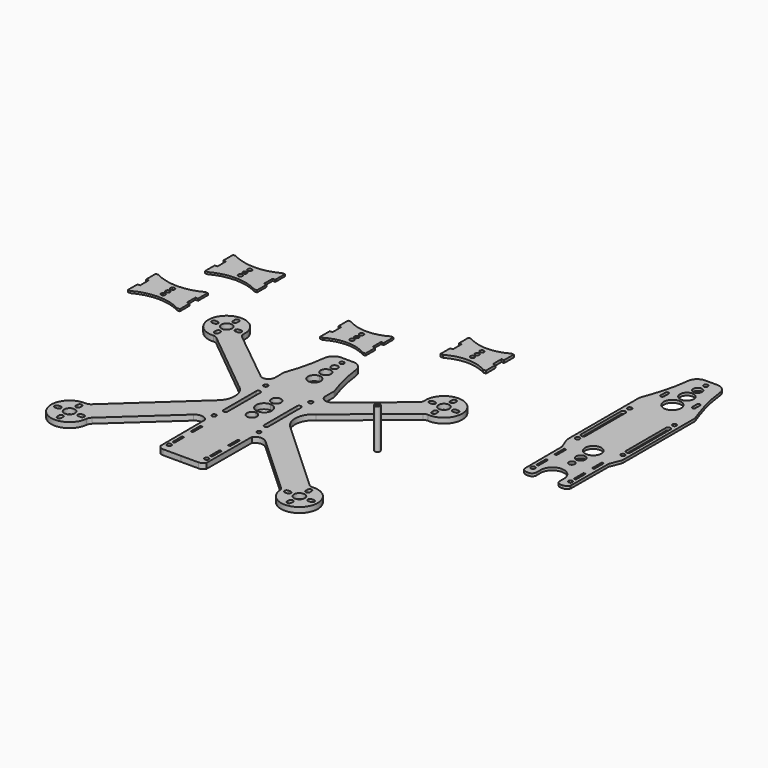
from build123d import *

# Parameters (mm, degrees)
F0_W      = 2
F0_H      = 9.1
F3_DEPTH  = 1.5
F4_W      = 2
F4_H      = 9.1
F5_DEPTH  = 2
F2_R      = 1.5875
F2_W      = 1.6002
F2_H      = 9.125
F6_DEPTH  = 2
F1_R      = 4
F1_R_2    = 1.5875
F7_DEPTH  = 4
F8_R      = 2
F8_R_2    = 1.3
F9_DEPTH  = 30
F10_W     = 2
F10_H     = 9.1
F11_DEPTH = 1.5
F12_W     = 2
F12_H     = 9.1
F13_DEPTH = 1.5


# Not quite as in the source:
# - ends of sketch curves that miss each other by under 0.0002 mm in the source are joined


with BuildPart() as f3:
    # F0 (on Top) → F3 (new body)
    with BuildSketch(Plane.XY):
        with BuildLine():
            Line((-44.4664459562, 44.7763409459), (-57.9039463685, 44.7763409459))
            Line((-57.9039463685, 44.7763409459), (-57.9039463685, 40.7740757426))
            Line((-57.9039463685, 40.7740757426), (-57.9039463685, 31.6763409459))
            ThreePointArc((-57.9039463685, 31.6763409459), (-42.9039463685, 35.7117386538), (-27.9039463685, 31.6763409459))
            Line((-27.9039463685, 31.6763409459), (-27.9039463685, 40.7740757426))
            Line((-27.9039463685, 40.7740757426), (-27.9039463685, 44.7763409459))
            Line((-27.9039463685, 44.7763409459), (-41.3414467807, 44.7763409459))
            ThreePointArc((-41.3414467807, 44.7763409459), (-41.7994933789, 43.6722203901), (-42.9039463685, 43.2149759459))
            ThreePointArc((-42.9039463685, 43.2149759459), (-44.0083993581, 43.6722203901), (-44.4664459562, 44.7763409459))
        make_face()
        with BuildLine():
            ThreePointArc((-42.9039463685, 38.8387946912), (-44.4664463685, 40.4012946912), (-42.9039463685, 41.9637946912))
            ThreePointArc((-42.9039463685, 41.9637946912), (-41.3414463685, 40.4012946912), (-42.9039463685, 38.8387946912))
        make_face(mode=Mode.SUBTRACT)
        with BuildLine():
            ThreePointArc((-27.9039463685, 57.8763409459), (-42.9039463685, 53.840943238), (-57.9039463685, 57.8763409459))
            Line((-57.9039463685, 57.8763409459), (-57.9039463685, 48.7763409459))
            Line((-57.9039463685, 48.7763409459), (-57.9039463685, 44.7763409459))
            Line((-57.9039463685, 44.7763409459), (-44.4664459562, 44.7763409459))
            ThreePointArc((-44.4664459562, 44.7763409459), (-44.0092019243, 45.8819289355), (-42.9039463685, 46.3399759459))
            ThreePointArc((-42.9039463685, 46.3399759459), (-41.7986908126, 45.8819289355), (-41.3414467807, 44.7763409459))
            Line((-41.3414467807, 44.7763409459), (-27.9039463685, 44.7763409459))
            Line((-27.9039463685, 44.7763409459), (-27.9039463685, 48.7763409459))
            Line((-27.9039463685, 48.7763409459), (-27.9039463685, 57.8763409459))
        make_face()
        with BuildLine():
            ThreePointArc((-42.9039463685, 50.8341467508), (-41.3414463685, 49.2716467508), (-42.9039463685, 47.7091467508))
            ThreePointArc((-42.9039463685, 47.7091467508), (-44.4664463685, 49.2716467508), (-42.9039463685, 50.8341467508))
        make_face(mode=Mode.SUBTRACT)
        with Locations((-26.9039463685, 53.3263409459)):
            Rectangle(F0_W, F0_H)
        Polygon((-25.9039463685, 40.7740757426), (-27.9039463685, 40.7740757426), (-27.9039463685, 31.6763409459), (-27.9039463685, 31.6740757426), (-25.9039463685, 31.6740757426), align=None)
        with Locations((-58.9039463685, 53.3263409459)):
            Rectangle(F0_W, F0_H)
        Polygon((-57.9039463685, 31.6763409459), (-57.9039463685, 40.7740757426), (-59.9039463685, 40.7740757426), (-59.9039463685, 31.6740757426), align=None)
    extrude(amount=F3_DEPTH)


with BuildPart() as f5:
    # F4 (on Top) → F5 (new body)
    with BuildSketch(Plane.XY):
        with BuildLine():
            ThreePointArc((41.3305214981, 84.1898763973), (26.3305214981, 80.1544786894), (11.3305214981, 84.1898763973))
            Line((11.3305214981, 84.1898763973), (11.3305214981, 75.0898763973))
            Line((11.3305214981, 75.0898763973), (11.3305214981, 71.0898763973))
            Line((11.3305214981, 71.0898763973), (24.7680219104, 71.0898763973))
            ThreePointArc((24.7680219104, 71.0898763973), (25.2252659423, 72.1954643869), (26.3305214981, 72.6535113973))
            ThreePointArc((26.3305214981, 72.6535113973), (27.435777054, 72.1954643869), (27.8930210859, 71.0898763973))
            Line((27.8930210859, 71.0898763973), (41.3305214981, 71.0898763973))
            Line((41.3305214981, 71.0898763973), (41.3305214981, 75.0898763973))
            Line((41.3305214981, 75.0898763973), (41.3305214981, 84.1898763973))
        make_face()
        with BuildLine():
            ThreePointArc((26.3305214981, 77.1476822022), (27.8930214981, 75.5851822022), (26.3305214981, 74.0226822022))
            ThreePointArc((26.3305214981, 74.0226822022), (24.7680214981, 75.5851822022), (26.3305214981, 77.1476822022))
        make_face(mode=Mode.SUBTRACT)
        with BuildLine():
            Line((24.7680219104, 71.0898763973), (11.3305214981, 71.0898763973))
            Line((11.3305214981, 71.0898763973), (11.3305214981, 67.087611194))
            Line((11.3305214981, 67.087611194), (11.3305214981, 57.9898763973))
            ThreePointArc((11.3305214981, 57.9898763973), (26.3305214981, 62.0252741052), (41.3305214981, 57.9898763973))
            Line((41.3305214981, 57.9898763973), (41.3305214981, 67.087611194))
            Line((41.3305214981, 67.087611194), (41.3305214981, 71.0898763973))
            Line((41.3305214981, 71.0898763973), (27.8930210859, 71.0898763973))
            ThreePointArc((27.8930210859, 71.0898763973), (27.4349744877, 69.9857558415), (26.3305214981, 69.5285113973))
            ThreePointArc((26.3305214981, 69.5285113973), (25.2260685085, 69.9857558415), (24.7680219104, 71.0898763973))
        make_face()
        with BuildLine():
            ThreePointArc((26.3305214981, 65.1523301426), (24.7680214981, 66.7148301426), (26.3305214981, 68.2773301426))
            ThreePointArc((26.3305214981, 68.2773301426), (27.8930214981, 66.7148301426), (26.3305214981, 65.1523301426))
        make_face(mode=Mode.SUBTRACT)
        Polygon((43.3305214981, 67.087611194), (41.3305214981, 67.087611194), (41.3305214981, 57.9898763973), (41.3305214981, 57.987611194), (43.3305214981, 57.987611194), align=None)
        with Locations((42.3305214981, 79.6398763973)):
            Rectangle(F4_W, F4_H)
        with Locations((10.3305214981, 79.6398763973)):
            Rectangle(F4_W, F4_H)
        Polygon((11.3305214981, 57.9898763973), (11.3305214981, 67.087611194), (9.3305214981, 67.087611194), (9.3305214981, 57.987611194), align=None)
    extrude(amount=F5_DEPTH)


with BuildPart() as f6:
    # F2 (on Top) → F6 (new body)
    with BuildSketch(Plane.XY):
        with BuildLine():
            Line((155.8763528676, 128.4774524202), (155.876246806, 128.4774524202))
            Line((155.876246806, 128.4774524202), (155.8761407443, 128.4774523998))
            Line((155.8761407443, 128.4774524202), (151.3094100886, 128.4774524202))
            ThreePointArc((151.3094100886, 128.4774524202), (146.4127010934, 126.6167403622), (143.9873656319, 121.9737072753))
            ThreePointArc((143.9873656319, 121.9737072753), (141.4366050173, 107.6108511655), (137.2573015197, 93.6347487897))
            Line((137.2573015197, 93.6347487897), (135.1935563122, 87.8591692184))
            ThreePointArc((135.1935563122, 87.8591692184), (135.0530988776, 87.3255692993), (135.0058168173, 86.7758224745))
            Line((135.0058168173, 86.7758224745), (135.0058168173, 19.9100591445))
            ThreePointArc((135.0058168173, 19.9100591445), (135.060963688, 19.3167136901), (135.2245151263, 18.743694552))
            Line((135.2245151263, 18.743694552), (138.1936514036, 11.1045397683))
            ThreePointArc((138.1936514036, 11.1045397683), (138.3556602367, 10.5396894348), (138.4123067823, 9.9548014711))
            Line((138.4123067823, 9.9548014711), (138.5925678775, -24.9512348722))
            ThreePointArc((138.5925678775, -24.9512348722), (140.1852851433, -26.826426264), (142.5436343491, -27.5273400025))
            Line((142.5436343491, -27.5273400025), (143.8996695078, -27.5273400025))
            ThreePointArc((143.8996695078, -27.5273400025), (146.1762594456, -26.5843455743), (147.1192538738, -24.3077556365))
            Line((147.1192538738, -24.3077556365), (147.1192538738, -20.6247556365))
            ThreePointArc((147.1192538738, -20.6247556365), (149.5794377566, -14.2301788079), (155.8897137171, -11.5611837055))
            ThreePointArc((155.8897137171, -11.5611837055), (162.2005028923, -14.2289650945), (164.6619166073, -20.6230686343))
            Line((164.6619166073, -20.6230686343), (164.6626249637, -24.3060685662))
            ThreePointArc((164.6626249637, -24.3060685662), (165.6060572341, -26.5824770945), (167.8828284972, -27.5250336456))
            Line((167.8828284972, -27.5250336456), (169.2388636308, -27.5247728375))
            ThreePointArc((169.2388636308, -27.5247728375), (171.5970779853, -26.8234055275), (173.1894345635, -24.9479078408))
            Line((173.1894345635, -24.9479078408), (173.3629821298, 9.9581625267))
            ThreePointArc((173.3629821298, 9.9581625267), (173.419516182, 10.5430613745), (173.5814163737, 11.1079428569))
            Line((173.5814163737, 11.1079428569), (176.5490833471, 18.7476685573))
            ThreePointArc((176.5490833471, 18.7476685573), (176.7125245728, 19.3207191409), (176.7675573235, 19.9140751908))
            Line((176.7675573235, 19.9140751908), (176.75469694, 86.7798372841))
            ThreePointArc((176.75469694, 86.7798372841), (176.707309147, 87.3295750049), (176.566749087, 87.8631478997))
            Line((176.566749087, 87.8631478997), (174.5018930926, 93.6383304413))
            ThreePointArc((174.5018930926, 93.6383304413), (170.3199016294, 107.6136287475), (167.7663786343, 121.9759940003))
            ThreePointArc((167.7663786343, 121.9759940003), (165.3401502168, 126.6185605332), (160.4430834388, 128.4783307661))
            Line((160.4430834388, 128.4783307661), (155.8763528676, 128.4774524405))
        make_face()
        with Locations((141.8560239264, -20.8835245555)):
            Circle(F2_R, mode=Mode.SUBTRACT)
        with Locations((141.8121739264, -12.3689241031)):
            Rectangle(F2_W, F2_H, mode=Mode.SUBTRACT)
        with Locations((141.8121739264, 4.7560758969)):
            Rectangle(F2_W, F2_H, mode=Mode.SUBTRACT)
        with Locations((138.9069576182, 24.590704959)):
            Circle(F2_R, mode=Mode.SUBTRACT)
        with BuildLine():
            ThreePointArc((137.3194112546, 67.0549892372), (139.055853514, 68.7740672747), (140.7575203822, 67.0205591086))
            Line((140.7575203822, 67.0205591086), (140.7578639328, 33.6104760546))
            Line((140.7578639328, 33.6104760546), (140.7578639328, 29.88865924))
            ThreePointArc((140.7578639328, 29.88865924), (139.0386515777, 28.1694424664), (137.3194303855, 29.8886504028))
            Line((137.3194303855, 29.8886504028), (137.3194112546, 33.6104406975))
            Line((137.3194112546, 33.6104406975), (137.3194112546, 67.0549892372))
        make_face(mode=Mode.SUBTRACT)
        with BuildLine():
            ThreePointArc((155.8890146168, -4.2914356483), (153.6566095072, -2.0721551798), (155.8885877383, 0.1475546091))
            ThreePointArc((155.8885877383, 0.1475546091), (158.1209928479, -2.0717258593), (155.8890146168, -4.2914356483))
        make_face(mode=Mode.SUBTRACT)
        with BuildLine():
            ThreePointArc((155.8883440274, 2.6818353952), (152.4370678505, 6.1205559329), (155.8876825898, 9.5599401956))
            ThreePointArc((155.8876825898, 9.5599401956), (159.3389587667, 6.1212196579), (155.8883440274, 2.6818353952))
        make_face(mode=Mode.SUBTRACT)
        with Locations((169.9251962268, -20.8808252644)):
            Circle(F2_R, mode=Mode.SUBTRACT)
        Polygon((170.7833763753, -7.7891995153), (170.7939351549, -16.9141934064), (169.1937362262, -16.9160450403), (169.1831774466, -7.7910511492), align=None, mode=Mode.SUBTRACT)
        Polygon((169.1633616547, 9.3339373861), (170.7635605834, 9.33578902), (170.774119363, 0.2107951289), (169.1739204343, 0.208943495), align=None, mode=Mode.SUBTRACT)
        with BuildLine():
            ThreePointArc((155.887452897, 11.9484512722), (149.8388017165, 17.9959392192), (155.8862896635, 24.0445903996))
            ThreePointArc((155.8862896635, 24.0445903996), (161.9349408439, 17.9971024527), (155.887452897, 11.9484512722))
        make_face(mode=Mode.SUBTRACT)
        with Locations((172.8655163598, 24.593970607)):
            Circle(F2_R, mode=Mode.SUBTRACT)
        with BuildLine():
            Line((174.4448954802, 67.0585594347), (174.4513279159, 33.6140115137))
            Line((174.4513279159, 33.6140115137), (174.452024602, 29.8922212841))
            ThreePointArc((174.452024602, 29.8922212841), (172.7331341001, 28.1726783007), (171.0135911167, 29.8915688027))
            Line((171.0135911167, 29.8915688027), (171.0128752946, 33.6133855484))
            Line((171.0128752946, 33.6133855484), (171.0067930382, 67.0234680505))
            ThreePointArc((171.0067930382, 67.0234680505), (172.7081226203, 68.7773034681), (174.4448954802, 67.0585594347))
        make_face(mode=Mode.SUBTRACT)
        with Locations((139.0386355169, 73.1351176697)):
            Circle(F2_R, mode=Mode.SUBTRACT)
        with BuildLine():
            ThreePointArc((145.2786560799, 101.8923559826), (145.2789936045, 101.8634246129), (145.2786560799, 101.8344932432))
            Line((145.2786560799, 101.8344932432), (145.2786560799, 97.5675112372))
            ThreePointArc((145.2786560799, 97.5675112372), (144.0533460411, 96.2985500188), (142.7987651392, 97.5385798675))
            Line((142.7987651392, 97.5385798675), (142.7987651392, 101.8634246129))
            ThreePointArc((142.7987651392, 101.8634246129), (144.0244127026, 103.1034544616), (145.2786560799, 101.8923559826))
        make_face(mode=Mode.SUBTRACT)
        with BuildLine():
            ThreePointArc((155.8803682862, 85.6193339205), (149.3345290592, 92.1782157718), (155.8791066864, 98.738356472))
            ThreePointArc((155.8791066864, 98.738356472), (162.4249459134, 92.1794746207), (155.8803682862, 85.6193339205))
        make_face(mode=Mode.SUBTRACT)
        with BuildLine():
            ThreePointArc((155.8789190085, 100.6899668871), (150.7560297607, 105.8118709374), (155.8779338109, 110.9347601852))
            ThreePointArc((155.8779338109, 110.9347601852), (161.0008230587, 105.8128561349), (155.8789190085, 100.6899668871))
        make_face(mode=Mode.SUBTRACT)
        with BuildLine():
            ThreePointArc((155.8777775383, 112.5597952039), (152.5637159996, 115.8732194059), (155.8771402016, 119.1872809446))
            ThreePointArc((155.8771402016, 119.1872809446), (159.1912017404, 115.8738567426), (155.8777775383, 112.5597952039))
        make_face(mode=Mode.SUBTRACT)
        with BuildLine():
            ThreePointArc((155.8776198499, 121.8899531092), (155.8768802972, 121.8899525924), (155.8761407443, 121.8899524202))
            ThreePointArc((155.8761407443, 121.8899524202), (154.2886407443, 123.4774524202), (155.8761407443, 125.0649524202))
            ThreePointArc((155.8761407443, 125.0649524202), (155.8765749713, 125.0649523608), (155.8770091982, 125.0649521826))
            ThreePointArc((155.8770091982, 125.0649521826), (157.464814495, 123.4777578591), (155.8776198499, 121.8899531092))
        make_face(mode=Mode.SUBTRACT)
        with Locations((172.7245018504, 73.1383570941)):
            Circle(F2_R, mode=Mode.SUBTRACT)
        with BuildLine():
            Line((166.4797822871, 97.569550058), (166.4789616126, 101.836531985))
            ThreePointArc((166.4789616126, 101.836531985), (166.4786185237, 101.8654632893), (166.4789504838, 101.8943947234))
            ThreePointArc((166.4789504838, 101.8943947234), (167.7329609058, 103.1057344103), (168.9588469431, 101.865940315))
            Line((168.9588469431, 101.865940315), (168.9596787464, 97.5410956496))
            ThreePointArc((168.9596787464, 97.5410956496), (167.7053363643, 96.3008245286), (166.4797822871, 97.569550058))
        make_face(mode=Mode.SUBTRACT)
    extrude(amount=F6_DEPTH)


with BuildPart() as f7:
    # F1 (on Top) → F7 (new body)
    with BuildSketch(Plane.XY):
        with BuildLine():
            Line((55.4423254621, -122.5938338167), (0.8312747552, -72.31776433))
            ThreePointArc((0.8312747552, -72.31776433), (-3.5713049649, -60.9524483755), (2.7441297756, -50.5280347721))
            Line((2.7441297756, -50.5280347721), (51.3242171863, -10.8932593465))
            ThreePointArc((51.3242171863, -10.8932593465), (52.7416112401, -10.1252404704), (54.3419180454, -9.9306202585))
            ThreePointArc((54.3419180454, -9.9306202585), (64.9351919977, 13.5546172758), (41.5501281912, 2.7420030758))
            ThreePointArc((41.5501281912, 2.7420030758), (41.2088558578, 0.7019316724), (39.9579419517, -0.945360814))
            Line((39.9579419517, -0.945360814), (0.7025146083, -32.6546178727))
            ThreePointArc((0.7025146083, -32.6546178727), (0.5270704544, -32.8033856058), (0.3447342931, -32.9436211712))
            ThreePointArc((0.3447342931, -32.9436211712), (-4.4980122119, -33.4435704761), (-7.3103707873, -29.4695571065))
            Line((-7.3103707873, -29.4695571065), (-7.3103707873, -21.2279371224))
            ThreePointArc((-7.3103707873, -21.2279371224), (-7.359671037, -20.6666688157), (-7.506061955, -20.1225894777))
            ThreePointArc((-7.506061955, -20.1225894777), (-11.7540587598, -6.0107609715), (-14.3386475919, 8.4981701128))
            ThreePointArc((-14.3386475919, 8.4981701128), (-16.7639830534, 13.1412031997), (-21.6606920486, 15.0019152577))
            Line((-21.6606920486, 15.0019152577), (-21.8785842975, 15.0019152577))
            Line((-21.8785842975, 15.0019152577), (-26.2273166427, 15.0019152577))
            Line((-26.2273166427, 15.0019152577), (-26.2274227043, 15.0019152577))
            Line((-26.2274227, 15.0019152577), (-26.2275287659, 15.0019152577))
            Line((-26.2275287659, 15.0019152578), (-30.5762611111, 15.0019211709))
            Line((-30.5762611111, 15.0019211709), (-30.7941533515, 15.0019214672))
            ThreePointArc((-30.7941533515, 15.0019214672), (-35.6908648767, 13.1412160673), (-38.1162066515, 8.4981862783))
            ThreePointArc((-38.1162066515, 8.4981862783), (-40.7008152117, -6.0107412918), (-44.9488312046, -20.1225640219))
            ThreePointArc((-44.9488312046, -20.1225640219), (-45.0952228624, -20.6666431607), (-45.1445238753, -21.2279114005))
            Line((-45.1445238753, -21.2279114005), (-45.1445350817, -29.4695313845))
            ThreePointArc((-45.1445350817, -29.4695313845), (-47.9568990637, -33.4435409315), (-52.7996448913, -32.9435850363))
            ThreePointArc((-52.7996448913, -32.9435850363), (-52.9819808591, -32.8033492249), (-53.157424808, -32.6545812554))
            Line((-53.1574248114, -32.6545812596), (-92.4128090441, -0.9452708203))
            ThreePointArc((-92.4128090441, -0.9452708203), (-93.6637207103, 0.7020233671), (-94.0049902698, 2.7420952345))
            ThreePointArc((-94.0049902698, 2.7420952345), (-117.3900393741, 13.5547412317), (-106.7967973552, -9.9305107065))
            ThreePointArc((-106.7967973552, -9.9305107065), (-105.1964908146, -10.1251330944), (-103.7790978051, -10.8931538978))
            Line((-103.7790978051, -10.8931538978), (-55.1990642866, -50.5279953787))
            ThreePointArc((-55.1990642866, -50.5279953787), (-48.8836437205, -60.9524175694), (-53.2862388943, -72.3177275376))
            Line((-53.2862388943, -72.3177275376), (-107.8973579627, -122.5937227683))
            ThreePointArc((-107.8973579627, -122.5937227683), (-109.6107464229, -123.6269577519), (-111.5920541618, -123.9056945287))
            ThreePointArc((-111.5920541618, -123.9056945287), (-122.9110206968, -146.5408303371), (-98.756834306, -138.9881052472))
            ThreePointArc((-98.756834306, -138.9881052472), (-98.2529376891, -137.2450612479), (-97.1601953583, -135.7966040057))
            Line((-97.1601953583, -135.7966040057), (-53.1895755998, -95.4842191234))
            ThreePointArc((-53.1895755998, -95.4842191234), (-48.3264853126, -93.815903761), (-43.7964935435, -96.2473843514))
            ThreePointArc((-43.7964935435, -96.2473843514), (-43.7450638141, -96.3412440629), (-43.7269025606, -96.446718379))
            Line((-43.7269025606, -96.446718379), (-43.51109813, -138.4267485338))
            ThreePointArc((-43.51109813, -138.4267485338), (-41.9183834139, -140.3019420913), (-39.5600351612, -141.0028590364))
            Line((-39.5600351612, -141.0028590364), (-26.2275287659, -141.0028771649))
            Line((-26.2275287659, -141.0028771649), (-12.8950223707, -141.0028771649))
            ThreePointArc((-12.8950223707, -141.0028771649), (-10.5366731649, -140.3019634265), (-8.9439558991, -138.4267720346))
            Line((-8.9439558991, -138.4267720346), (-8.7280943872, -96.4467421734))
            ThreePointArc((-8.7280943872, -96.4467421734), (-8.7099329903, -96.3412678819), (-8.6585031333, -96.2474082404))
            ThreePointArc((-8.6585031333, -96.2474082404), (-4.1285080581, -93.8159338094), (0.7345799607, -95.4842557844))
            Line((0.7345799607, -95.4842557844), (44.7051449055, -135.7967004544))
            ThreePointArc((44.7051449055, -135.7967004544), (45.7978852668, -137.2451591825), (46.3017795137, -138.988203867))
            ThreePointArc((46.3017795137, -138.988203867), (70.4559556348, -146.5409617999), (59.1370198774, -123.9058106008))
            ThreePointArc((59.1370198774, -123.9058106008), (57.1557125175, -123.62707113), (55.4423254621, -122.5938338167))
        make_face()
        with BuildLine():
            Line((-114.039597116, -147.1295236826), (-114.0395949405, -145.5295236826))
            ThreePointArc((-114.0395949405, -145.5295236826), (-112.4395927649, -143.9295258581), (-110.8395949405, -145.5295280337))
            Line((-110.8395949405, -145.5295280337), (-110.839597116, -147.1295280337))
            ThreePointArc((-110.839597116, -147.1295280337), (-112.4395992916, -148.7295258581), (-114.039597116, -147.1295236826))
        make_face(mode=Mode.SUBTRACT)
        with BuildLine():
            ThreePointArc((-122.0395863742, -139.2295128048), (-123.6395841987, -137.6295106292), (-122.0395820231, -136.0295128048))
            Line((-122.0395820231, -136.0295128048), (-120.4395820231, -136.0295149804))
            ThreePointArc((-120.4395820231, -136.0295149804), (-118.8395841987, -137.6295171559), (-120.4395863742, -139.2295149803))
            Line((-120.4395863742, -139.2295149803), (-122.0395863742, -139.2295128048))
        make_face(mode=Mode.SUBTRACT)
        with Locations((-112.4395841987, -137.6295258581)):
            Circle(F1_R, mode=Mode.SUBTRACT)
        with BuildLine():
            ThreePointArc((-104.4395863742, -139.2295367359), (-106.0395841987, -137.6295345604), (-104.4395820231, -136.0295367359))
            Line((-104.4395820231, -136.0295367359), (-102.8395820231, -136.0295389115))
            ThreePointArc((-102.8395820231, -136.0295389115), (-101.2395841987, -137.629541087), (-102.8395863742, -139.2295389115))
            Line((-102.8395863742, -139.2295389115), (-104.4395863742, -139.2295367359))
        make_face(mode=Mode.SUBTRACT)
        with BuildLine():
            ThreePointArc((-114.0395712813, -128.1295236826), (-112.4395691057, -126.5295258581), (-110.8395712813, -128.1295280337))
            Line((-110.8395712813, -128.1295280337), (-110.8395734569, -129.7295280337))
            ThreePointArc((-110.8395734569, -129.7295280337), (-112.4395756324, -131.3295258581), (-114.0395734569, -129.7295236826))
            Line((-114.0395734569, -129.7295236826), (-114.0395712813, -128.1295236826))
        make_face(mode=Mode.SUBTRACT)
        with Locations((-40.2476365481, -134.3575674396)):
            Circle(F1_R_2, mode=Mode.SUBTRACT)
        Polygon((-39.4913811763, -130.4069432304), (-41.0915811763, -130.4069410545), (-41.0915687689, -121.2819410546), (-39.4913687689, -121.2819432304), align=None, mode=Mode.SUBTRACT)
        Polygon((-39.4913578911, -113.2819432304), (-41.0915578911, -113.2819410546), (-41.0915454836, -104.1569410546), (-39.4913454836, -104.1569432304), align=None, mode=Mode.SUBTRACT)
        with Locations((-43.064958687, -88.83576076)):
            Circle(F1_R_2, mode=Mode.SUBTRACT)
        with Locations((-12.207411948, -134.357586503)):
            Circle(F1_R_2, mode=Mode.SUBTRACT)
        Polygon((-11.363488763, -121.2819410546), (-11.3634763555, -130.4069410545), (-12.9636763555, -130.4069432304), (-12.963688763, -121.2819432304), align=None, mode=Mode.SUBTRACT)
        with BuildLine():
            Line((58.3845312536, -147.1296430826), (58.3845312536, -145.5296430826))
            ThreePointArc((58.3845312536, -145.5296430826), (59.9845312536, -143.9296430826), (61.5845312536, -145.5296430826))
            Line((61.5845312536, -145.5296430826), (61.5845312536, -147.1296430826))
            ThreePointArc((61.5845312536, -147.1296430826), (59.9845312536, -148.7296430826), (58.3845312536, -147.1296430826))
        make_face(mode=Mode.SUBTRACT)
        with BuildLine():
            Line((50.3845312536, -136.0296430826), (51.9845312536, -136.0296430826))
            ThreePointArc((51.9845312536, -136.0296430826), (53.5845312536, -137.6296430826), (51.9845312536, -139.2296430826))
            Line((51.9845312536, -139.2296430826), (50.3845312536, -139.2296430826))
            ThreePointArc((50.3845312536, -139.2296430826), (48.7845312536, -137.6296430826), (50.3845312536, -136.0296430826))
        make_face(mode=Mode.SUBTRACT)
        with Locations((59.9845312536, -137.6296430826)):
            Circle(F1_R, mode=Mode.SUBTRACT)
        with BuildLine():
            Line((67.9845312536, -136.0296430826), (69.5845312536, -136.0296430826))
            ThreePointArc((69.5845312536, -136.0296430826), (71.1845312536, -137.6296430826), (69.5845312536, -139.2296430826))
            Line((69.5845312536, -139.2296430826), (67.9845312536, -139.2296430826))
            ThreePointArc((67.9845312536, -139.2296430826), (66.3845312536, -137.6296430826), (67.9845312536, -136.0296430826))
        make_face(mode=Mode.SUBTRACT)
        with BuildLine():
            Line((61.5845312536, -128.1296430826), (61.5845312536, -129.7296430826))
            ThreePointArc((61.5845312536, -129.7296430826), (59.9845312536, -131.3296430826), (58.3845312536, -129.7296430826))
            Line((58.3845312536, -129.7296430826), (58.3845312536, -128.1296430826))
            ThreePointArc((58.3845312536, -128.1296430826), (59.9845312536, -126.5296430826), (61.5845312536, -128.1296430826))
        make_face(mode=Mode.SUBTRACT)
        Polygon((-11.3635120482, -104.1569410546), (-11.3634996407, -113.2819410546), (-12.9636996407, -113.2819432304), (-12.9637120482, -104.1569432304), align=None, mode=Mode.SUBTRACT)
        with Locations((-9.390027912, -88.8357836543)):
            Circle(F1_R_2, mode=Mode.SUBTRACT)
        with BuildLine():
            ThreePointArc((-26.2274859928, -78.0884044908), (-29.9104989964, -74.4054019869), (-26.2274809849, -70.7224044909))
            ThreePointArc((-26.2274809849, -70.7224044909), (-22.5444679813, -74.4054069948), (-26.2274859928, -78.0884044908))
        make_face(mode=Mode.SUBTRACT)
        with BuildLine():
            Line((-43.0649509726, -79.9457608638), (-43.0608459045, -49.4593622105))
            ThreePointArc((-43.0608459045, -49.4593622105), (-43.0649093649, -49.3456362447), (-43.0608152777, -49.2319113774))
            ThreePointArc((-43.0608152777, -49.2319113774), (-41.4782727262, -47.7583502402), (-39.8941283465, -49.2301892044))
            ThreePointArc((-39.8941283465, -49.2301892044), (-39.8899093793, -49.3458521643), (-39.894128661, -49.4615151127))
            Line((-39.8941286549, -49.4615151127), (-39.894169948, -79.830313823))
            ThreePointArc((-39.8941699542, -79.830313823), (-41.4196889346, -81.5324234246), (-43.0649509726, -79.9457608638))
        make_face(mode=Mode.SUBTRACT)
        with Locations((-43.0648927468, -40.3403965985)):
            Circle(F1_R_2, mode=Mode.SUBTRACT)
        with BuildLine():
            Line((-106.1135999626, -4.112378486), (-106.1136021381, -5.712378486))
            ThreePointArc((-106.1136021381, -5.712378486), (-107.7136043137, -7.3123763104), (-109.3136021381, -5.7123741349))
            Line((-109.3136021381, -5.7123741349), (-109.3135999626, -4.1123741349))
            ThreePointArc((-109.3135999626, -4.1123741349), (-107.713597787, -2.5123763104), (-106.1135999626, -4.112378486))
        make_face(mode=Mode.SUBTRACT)
        with BuildLine():
            ThreePointArc((-115.7135870452, 5.3876345673), (-114.1135892208, 3.7876323918), (-115.7135913963, 2.1876345674))
            Line((-115.7135913963, 2.1876345674), (-117.3135913963, 2.1876367429))
            ThreePointArc((-117.3135913963, 2.1876367429), (-118.9135892208, 3.7876389185), (-117.3135870452, 5.3876367429))
            Line((-117.3135870452, 5.3876367429), (-115.7135870452, 5.3876345673))
        make_face(mode=Mode.SUBTRACT)
        with Locations((-107.7135892208, 3.7876236896)):
            Circle(F1_R, mode=Mode.SUBTRACT)
        with BuildLine():
            Line((-109.313578479, 11.6876258651), (-109.3135763034, 13.2876258651))
            ThreePointArc((-109.3135763034, 13.2876258651), (-107.7135741278, 14.8876236896), (-106.1135763034, 13.287621514))
            Line((-106.1135763034, 13.287621514), (-106.113578479, 11.687621514))
            ThreePointArc((-106.113578479, 11.687621514), (-107.7135806545, 10.0876236896), (-109.313578479, 11.6876258651))
        make_face(mode=Mode.SUBTRACT)
        with BuildLine():
            Line((-98.1135913963, 2.1876106362), (-99.7135913963, 2.1876128118))
            ThreePointArc((-99.7135913963, 2.1876128118), (-101.3135892208, 3.7876149873), (-99.7135870452, 5.3876128118))
            Line((-99.7135870452, 5.3876128118), (-98.1135870452, 5.3876106362))
            ThreePointArc((-98.1135870452, 5.3876106362), (-96.5135892208, 3.7876084607), (-98.1135913963, 2.1876106362))
        make_face(mode=Mode.SUBTRACT)
        with BuildLine():
            ThreePointArc((-26.2274717449, -57.1313950416), (-20.358389823, -63.0004849438), (-26.2274797253, -68.8695668657))
            ThreePointArc((-26.2274797253, -68.8695668657), (-32.0965616472, -63.0004769635), (-26.2274717449, -57.1313950416))
        make_face(mode=Mode.SUBTRACT)
        with BuildLine():
            ThreePointArc((-9.3941174711, -49.2319342661), (-9.3900235385, -49.345659139), (-9.3940871535, -49.4593850992))
            Line((-9.3940871535, -49.4593850992), (-9.3900235385, -79.9457837581))
            ThreePointArc((-9.3900235385, -79.9457837581), (-11.0352877339, -81.5324440818), (-12.5608044, -79.8303324059))
            Line((-12.5608044, -79.8303324059), (-12.5608044, -49.4615336956))
            ThreePointArc((-12.5608044, -49.4615336956), (-12.5650235244, -49.3458707412), (-12.5608044, -49.2302077868))
            ThreePointArc((-12.5608044, -49.2302077868), (-10.9766580187, -47.7583709771), (-9.3941174711, -49.2319342661))
        make_face(mode=Mode.SUBTRACT)
        with BuildLine():
            ThreePointArc((-26.2274654774, -47.9125574164), (-22.5444679813, -51.5955599203), (-26.2274704853, -55.2785574164))
            ThreePointArc((-26.2274704853, -55.2785574164), (-29.9104679813, -51.5955549125), (-26.2274654774, -47.9125574164))
        make_face(mode=Mode.SUBTRACT)
        with Locations((-9.390027912, -40.3404194927)):
            Circle(F1_R_2, mode=Mode.SUBTRACT)
        with BuildLine():
            ThreePointArc((-26.2274404616, -11.1171243326), (-21.4699158383, -15.8746554248), (-26.2274469305, -20.6321800481))
            ThreePointArc((-26.2274469305, -20.6321800481), (-30.9849715539, -15.8746489559), (-26.2274404616, -11.1171243326))
        make_face(mode=Mode.SUBTRACT)
        with BuildLine():
            ThreePointArc((-26.2274337429, -1.2346663439), (-22.3490281693, -5.1130771911), (-26.2274390165, -8.9914827647))
            ThreePointArc((-26.2274390165, -8.9914827647), (-30.1058445901, -5.1130719176), (-26.2274337429, -1.2346663439))
        make_face(mode=Mode.SUBTRACT)
        with BuildLine():
            ThreePointArc((-26.227429149, 5.5224765168), (-23.7401115453, 3.0351555311), (-26.2274325311, 0.5478379274))
            ThreePointArc((-26.2274325311, 0.5478379274), (-28.7147501347, 3.0351589131), (-26.227429149, 5.5224765168))
        make_face(mode=Mode.SUBTRACT)
        with BuildLine():
            ThreePointArc((-26.2273255998, 8.4144152707), (-26.2274271829, 8.4144152609), (-26.2275287659, 8.4144152577))
            ThreePointArc((-26.2275287659, 8.4144152708), (-27.8148234413, 10.0019152575), (-26.2275287659, 11.5894152443))
            ThreePointArc((-26.2275287659, 11.5894152577), (-26.2274250243, 11.5894152543), (-26.2273212827, 11.5894152441))
            ThreePointArc((-26.2273212827, 11.5894152441), (-24.6400287659, 10.0019130991), (-26.2273255998, 8.4144152707))
        make_face(mode=Mode.SUBTRACT)
        with BuildLine():
            Line((53.6587285638, -5.712487109), (53.6587285638, -4.112487109))
            ThreePointArc((53.6587285638, -4.112487109), (55.2587285638, -2.512487109), (56.8587285638, -4.112487109))
            Line((56.8587285638, -4.112487109), (56.8587285638, -5.712487109))
            ThreePointArc((56.8587285638, -5.712487109), (55.2587285638, -7.312487109), (53.6587285638, -5.712487109))
        make_face(mode=Mode.SUBTRACT)
        with BuildLine():
            Line((45.6587285638, 5.387512891), (47.2587285638, 5.387512891))
            ThreePointArc((47.2587285638, 5.387512891), (48.8587285638, 3.787512891), (47.2587285638, 2.187512891))
            Line((47.2587285638, 2.187512891), (45.6587285638, 2.187512891))
            ThreePointArc((45.6587285638, 2.187512891), (44.0587285638, 3.787512891), (45.6587285638, 5.387512891))
        make_face(mode=Mode.SUBTRACT)
        with Locations((55.2587285638, 3.787512891)):
            Circle(F1_R, mode=Mode.SUBTRACT)
        with BuildLine():
            Line((63.2587285638, 5.387512891), (64.8587285638, 5.387512891))
            ThreePointArc((64.8587285638, 5.387512891), (66.4587285638, 3.787512891), (64.8587285638, 2.187512891))
            Line((64.8587285638, 2.187512891), (63.2587285638, 2.187512891))
            ThreePointArc((63.2587285638, 2.187512891), (61.6587285638, 3.787512891), (63.2587285638, 5.387512891))
        make_face(mode=Mode.SUBTRACT)
        with BuildLine():
            Line((56.8587285638, 13.287512891), (56.8587285638, 11.687512891))
            ThreePointArc((56.8587285638, 11.687512891), (55.2587285638, 10.087512891), (53.6587285638, 11.687512891))
            Line((53.6587285638, 11.687512891), (53.6587285638, 13.287512891))
            ThreePointArc((53.6587285638, 13.287512891), (55.2587285638, 14.887512891), (56.8587285638, 13.287512891))
        make_face(mode=Mode.SUBTRACT)
    extrude(amount=F7_DEPTH)


with BuildPart() as f9:
    # F8 (on Top) → F9 (new body)
    with BuildSketch(Plane.XY):
        with Locations((54.602060467, -57.8380823135)):
            Circle(F8_R)
        with Locations((54.602060467, -57.8380823135)):
            Circle(F8_R_2, mode=Mode.SUBTRACT)
    extrude(amount=F9_DEPTH)


with BuildPart() as f11:
    # F10 (on Top) → F11 (new body)
    with BuildSketch(Plane.XY):
        with BuildLine():
            ThreePointArc((-127.6205689662, 80.8045635421), (-136.1038902285, 77.5559695059), (-145.1205339662, 76.451325418))
            Line((-145.1205339662, 76.451325418), (-145.1205339662, 73.762369347))
            ThreePointArc((-145.1205339662, 73.762369347), (-143.5580339662, 72.199869347), (-145.1205339662, 70.637369347))
            Line((-145.1205339662, 70.637369347), (-145.1205339662, 69.2681985421))
            ThreePointArc((-145.1205339662, 69.2681985421), (-144.0152784103, 68.8101515317), (-143.5580343784, 67.7045635421))
            Line((-143.5580343784, 67.7045635421), (-127.6205689662, 67.7045635421))
            Line((-127.6205689662, 67.7045635421), (-127.6205689662, 71.7045635421))
            Line((-127.6205689662, 71.7045635421), (-127.6205689662, 80.8045635421))
        make_face()
        with Locations((-163.6204989662, 76.2545635421)):
            Rectangle(F10_W, F10_H)
        with BuildLine():
            ThreePointArc((-145.1205339662, 76.451325418), (-154.1371777038, 77.5559695059), (-162.6204989662, 80.8045635421))
            Line((-162.6204989662, 80.8045635421), (-162.6204989662, 71.7045635421))
            Line((-162.6204989662, 71.7045635421), (-162.6204989662, 67.7045635421))
            Line((-162.6204989662, 67.7045635421), (-146.6830335539, 67.7045635421))
            ThreePointArc((-146.6830335539, 67.7045635421), (-146.225789522, 68.8101515317), (-145.1205339662, 69.2681985421))
            Line((-145.1205339662, 69.2681985421), (-145.1205339662, 70.637369347))
            ThreePointArc((-145.1205339662, 70.637369347), (-146.6830339662, 72.199869347), (-145.1205339662, 73.762369347))
            Line((-145.1205339662, 73.762369347), (-145.1205339662, 76.451325418))
        make_face()
        with BuildLine():
            ThreePointArc((-143.5580343784, 67.7045635421), (-144.0160809766, 66.6004429862), (-145.1205339662, 66.1431985421))
            Line((-145.1205339662, 66.1431985421), (-145.1205339662, 64.8920172874))
            ThreePointArc((-145.1205339662, 64.8920172874), (-143.5580339662, 63.3295172874), (-145.1205339662, 61.7670172874))
            Line((-145.1205339662, 61.7670172874), (-145.1205339662, 58.9812437579))
            ThreePointArc((-145.1205339662, 58.9812437579), (-136.1010535943, 57.8704791393), (-127.6205689662, 54.6045635421))
            Line((-127.6205689662, 54.6045635421), (-127.6205689662, 63.7022983387))
            Line((-127.6205689662, 63.7022983387), (-127.6205689662, 67.7045635421))
            Line((-127.6205689662, 67.7045635421), (-143.5580343784, 67.7045635421))
        make_face()
        Polygon((-125.6205689662, 63.7022983387), (-127.6205689662, 63.7022983387), (-127.6205689662, 54.6045635421), (-127.6205689662, 54.6022983387), (-125.6205689662, 54.6022983387), align=None)
        with Locations((-126.6205689662, 76.2545635421)):
            Rectangle(F10_W, F10_H)
        Polygon((-162.6204989662, 54.6045635421), (-162.6204989662, 63.7022983387), (-164.6204989662, 63.7022983387), (-164.6204989662, 54.6022983387), align=None)
        with BuildLine():
            Line((-146.6830335539, 67.7045635421), (-162.6204989662, 67.7045635421))
            Line((-162.6204989662, 67.7045635421), (-162.6204989662, 63.7022983387))
            Line((-162.6204989662, 63.7022983387), (-162.6204989662, 54.6045635421))
            ThreePointArc((-162.6204989662, 54.6045635421), (-154.140014338, 57.8704791393), (-145.1205339662, 58.9812437579))
            Line((-145.1205339662, 58.9812437579), (-145.1205339662, 61.7670172874))
            ThreePointArc((-145.1205339662, 61.7670172874), (-146.6830339662, 63.3295172874), (-145.1205339662, 64.8920172874))
            Line((-145.1205339662, 64.8920172874), (-145.1205339662, 66.1431985421))
            ThreePointArc((-145.1205339662, 66.1431985421), (-146.2249869558, 66.6004429862), (-146.6830335539, 67.7045635421))
        make_face()
    extrude(amount=F11_DEPTH)


with BuildPart() as f13:
    # F12 (on Top) → F13 (new body)
    with BuildSketch(Plane.XY):
        with BuildLine():
            ThreePointArc((-147.9669716612, 33.8699137749), (-156.4502929235, 30.6213197387), (-165.4669366612, 29.5166756508))
            Line((-165.4669366612, 29.5166756508), (-165.4669366612, 26.8277195798))
            ThreePointArc((-165.4669366612, 26.8277195798), (-163.9044366612, 25.2652195798), (-165.4669366612, 23.7027195798))
            Line((-165.4669366612, 23.7027195798), (-165.4669366612, 22.3335487749))
            ThreePointArc((-165.4669366612, 22.3335487749), (-164.3616811053, 21.8755017645), (-163.9044370734, 20.7699137749))
            Line((-163.9044370734, 20.7699137749), (-147.9669716612, 20.7699137749))
            Line((-147.9669716612, 20.7699137749), (-147.9669716612, 24.7699137749))
            Line((-147.9669716612, 24.7699137749), (-147.9669716612, 33.8699137749))
        make_face()
        with BuildLine():
            ThreePointArc((-165.4669366612, 29.5166756508), (-174.4835803988, 30.6213197387), (-182.9669016612, 33.8699137749))
            Line((-182.9669016612, 33.8699137749), (-182.9669016612, 24.7699137749))
            Line((-182.9669016612, 24.7699137749), (-182.9669016612, 20.7699137749))
            Line((-182.9669016612, 20.7699137749), (-167.0294362489, 20.7699137749))
            ThreePointArc((-167.0294362489, 20.7699137749), (-166.572192217, 21.8755017645), (-165.4669366612, 22.3335487749))
            Line((-165.4669366612, 22.3335487749), (-165.4669366612, 23.7027195798))
            ThreePointArc((-165.4669366612, 23.7027195798), (-167.0294366612, 25.2652195798), (-165.4669366612, 26.8277195798))
            Line((-165.4669366612, 26.8277195798), (-165.4669366612, 29.5166756508))
        make_face()
        with BuildLine():
            Line((-167.0294362489, 20.7699137749), (-182.9669016612, 20.7699137749))
            Line((-182.9669016612, 20.7699137749), (-182.9669016612, 16.7676485716))
            Line((-182.9669016612, 16.7676485716), (-182.9669016612, 7.6699137749))
            ThreePointArc((-182.9669016612, 7.6699137749), (-174.486417033, 10.9358293721), (-165.4669366612, 12.0465939907))
            Line((-165.4669366612, 12.0465939907), (-165.4669366612, 14.8323675202))
            ThreePointArc((-165.4669366612, 14.8323675202), (-167.0294366612, 16.3948675202), (-165.4669366612, 17.9573675202))
            Line((-165.4669366612, 17.9573675202), (-165.4669366612, 19.2085487749))
            ThreePointArc((-165.4669366612, 19.2085487749), (-166.5713896508, 19.6657932191), (-167.0294362489, 20.7699137749))
        make_face()
        Polygon((-182.9669016612, 7.6699137749), (-182.9669016612, 16.7676485716), (-184.9669016612, 16.7676485716), (-184.9669016612, 7.6676485716), align=None)
        Polygon((-145.9669716612, 16.7676485716), (-147.9669716612, 16.7676485716), (-147.9669716612, 7.6699137749), (-147.9669716612, 7.6676485716), (-145.9669716612, 7.6676485716), align=None)
        with Locations((-146.9669716612, 29.3199137749)):
            Rectangle(F12_W, F12_H)
        with Locations((-183.9669016612, 29.3199137749)):
            Rectangle(F12_W, F12_H)
        with BuildLine():
            ThreePointArc((-163.9044370734, 20.7699137749), (-164.3624836715, 19.6657932191), (-165.4669366612, 19.2085487749))
            Line((-165.4669366612, 19.2085487749), (-165.4669366612, 17.9573675202))
            ThreePointArc((-165.4669366612, 17.9573675202), (-163.9044366612, 16.3948675202), (-165.4669366612, 14.8323675202))
            Line((-165.4669366612, 14.8323675202), (-165.4669366612, 12.0465939907))
            ThreePointArc((-165.4669366612, 12.0465939907), (-156.4474562893, 10.9358293721), (-147.9669716612, 7.6699137749))
            Line((-147.9669716612, 7.6699137749), (-147.9669716612, 16.7676485716))
            Line((-147.9669716612, 16.7676485716), (-147.9669716612, 20.7699137749))
            Line((-147.9669716612, 20.7699137749), (-163.9044370734, 20.7699137749))
        make_face()
    extrude(amount=F13_DEPTH)


solid = Compound([f3.part, f5.part, f6.part, f7.part, f9.part, f11.part, f13.part])
